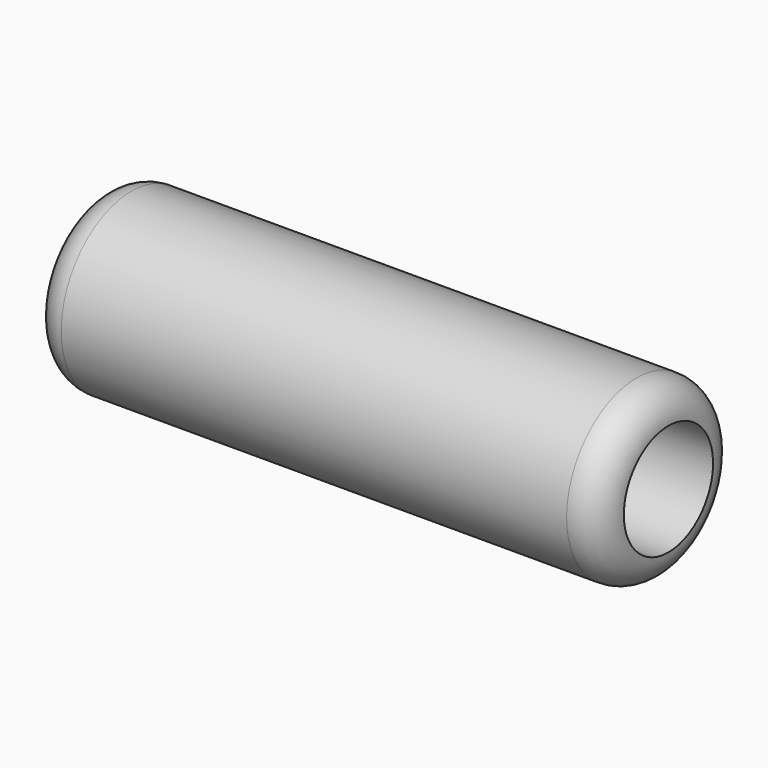
from build123d import *


# Not quite as in the source:
# - a fillet or chamfer that OpenCascade refuses, or shapes differently, is made with other operations: its cross-section is extruded or revolved along the edge and cut away or added


with BuildPart() as f1:
    # F0 (on Front) → F1 (revolve)
    with BuildSketch(Plane.XZ):
        Polygon((7.3269232676, 0), (0, 0), (0, -17.4752), (113.5126, -17.4752), (113.5126, -11.1252), (7.3269232676, -11.1252), align=None)
    revolve(axis=Axis((18.5955958441, 0, 0), (1, 0, 0)))

    # F2: fillet of radius 6.35 on 2 edges, made by hand

    # F2_s1 → F2_t2 (revolve, cut)
    with BuildSketch(Plane.XZ):
        with BuildLine():
            ThreePointArc((0, -11.1252), (1.8598719395, -15.6153280605), (6.35, -17.4752))
            Line((6.35, -17.4752), (0, -17.4752))
            Line((0, -17.4752), (0, -11.1252))
        make_face()
    revolve(axis=Axis((0, 0, 0), (1, 0, 0)), mode=Mode.SUBTRACT)

    # F2_s3 → F2_t4 (revolve, cut)
    with BuildSketch(Plane.XZ):
        with BuildLine():
            ThreePointArc((107.1626, -17.4752), (111.6527280605, -15.6153280605), (113.5126, -11.1252))
            Line((113.5126, -11.1252), (113.5126, -17.4752))
            Line((113.5126, -17.4752), (107.1626, -17.4752))
        make_face()
    revolve(axis=Axis((113.5126, 0, 0), (1, 0, 0)), mode=Mode.SUBTRACT)


solid = f1.part
